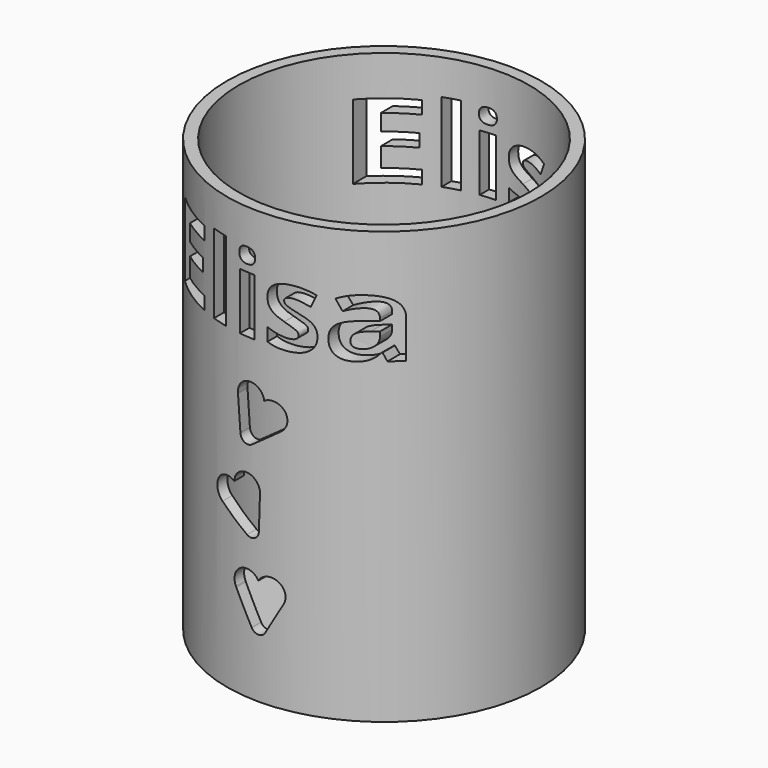
from build123d import *

# Parameters (mm, degrees)
F0_R         = 40
F1_DEPTH     = 110
F2_R         = 37
F3_DEPTH     = 104
F4_TEXT_SIZE = 26.5376641327
F5_DEPTH     = 45
F6_DEPTH     = 45


# Not quite as in the source:
# - Text() gives the source's letters only with a copy of the font that has no kerning and outlines rounded to 1/6400 em; it was checked with that copy


with BuildPart() as f1:
    # F0 (on Top) → F1 (new body)
    with BuildSketch(Plane.XY):
        Circle(F0_R)
    extrude(amount=F1_DEPTH)

    # F2 (on face) → F3 (cut)
    with BuildSketch(Plane.XY.offset(110)):
        Circle(F2_R)
    extrude(amount=-F3_DEPTH, mode=Mode.SUBTRACT)

    # F4 (on Front) → F5 (cut, symmetric)
    with BuildSketch(Plane.XZ):
        with BuildLine():
            ThreePointArc((6.0980562795, 23.7189958695), (4.7163435964, 28.3977795102), (0, 27.1502822652))
            ThreePointArc((0, 27.1502822652), (-4.7163435964, 28.3977795102), (-6.0980562795, 23.7189958695))
            Line((-6.0980562795, 23.7189958695), (-5.9870867882, 23.523414382))
            Line((-5.9870867882, 23.523414382), (-1.7395100946, 16.03714624))
            ThreePointArc((-1.7395100946, 16.03714624), (-1.0064952106, 15.2958291084), (0, 15.024113631))
            ThreePointArc((0, 15.024113631), (1.0064952106, 15.2958291084), (1.7395100946, 16.03714624))
            Line((1.7395100946, 16.03714624), (5.9870867882, 23.523414382))
            Line((5.9870867882, 23.523414382), (6.0980562795, 23.7189958695))
        make_face()
        with BuildLine():
            Line((-5.9870867882, 23.523414382), (-6.0980562795, 23.7189958695))
            ThreePointArc((-6.0980562795, 23.7189958695), (-6.0441426655, 23.6203136933), (-5.9870867882, 23.523414382))
        make_face()
        with BuildLine():
            ThreePointArc((5.9870867882, 23.523414382), (6.0441426655, 23.6203136933), (6.0980562795, 23.7189958695))
            Line((6.0980562795, 23.7189958695), (5.9870867882, 23.523414382))
        make_face()
        with BuildLine():
            ThreePointArc((0.3949105078, 46.6853627057), (-2.8839636057, 50.4050689505), (-6.5919721438, 47.1129719469))
            ThreePointArc((-6.5919721438, 47.1129719469), (-11.4072011799, 45.9294182599), (-10.2065108138, 41.1184336783))
            Line((-10.2065108138, 41.1184336783), (-2.9654370981, 36.4651584979))
            ThreePointArc((-2.9654370981, 36.4651584979), (-1.9718103227, 36.1496149336), (-0.9543788911, 36.3769806997))
            ThreePointArc((-0.9543788911, 36.3769806997), (-0.1895946703, 37.0854769985), (0.1147386299, 38.0825944199))
            Line((0.1147386299, 38.0825944199), (0.3949105078, 46.6853627057))
        make_face()
        with BuildLine():
            ThreePointArc((5.5303396509, 62.2585198994), (6.255422096, 67.0828749592), (1.453748051, 67.9454714242))
            ThreePointArc((1.453748051, 67.9454714242), (-2.2934957595, 71.0693008242), (-5.523092133, 67.4128197891))
            Line((-5.523092133, 67.4128197891), (-5.5051759271, 67.1886650304))
            Line((-5.5051759271, 67.1886650304), (-4.8193977228, 58.6086984387))
            ThreePointArc((-4.8193977228, 58.6086984387), (-4.468354783, 57.6270514736), (-3.6709922587, 56.9554303641))
            ThreePointArc((-3.6709922587, 56.9554303641), (-2.643965889, 56.7763249608), (-1.6663346341, 57.1384009738))
            Line((-1.6663346341, 57.1384009738), (5.3471108284, 62.1281606078))
            Line((5.3471108284, 62.1281606078), (5.5303396509, 62.2585198994))
        make_face()
        with BuildLine():
            Line((-5.5051759271, 67.1886650304), (-5.523092133, 67.4128197891))
            ThreePointArc((-5.523092133, 67.4128197891), (-5.5159346946, 67.3005984865), (-5.5051759271, 67.1886650304))
        make_face()
        with BuildLine():
            ThreePointArc((5.3471108284, 62.1281606078), (5.4397724329, 62.1918683525), (5.5303396509, 62.2585198994))
            Line((5.5303396509, 62.2585198994), (5.3471108284, 62.1281606078))
        make_face()
        with Locations((-30, 80.8928818245)):
            Text('Elisa', F4_TEXT_SIZE, font='Open Sans', font_style=FontStyle.BOLD, text_align=(TextAlign.LEFT, TextAlign.BOTTOM))
    extrude(amount=F5_DEPTH, both=True, mode=Mode.SUBTRACT)

    # F4 (on Front) → F6 (cut, symmetric)
    with BuildSketch(Plane.XZ):
        with BuildLine():
            ThreePointArc((6.0980562795, 23.7189958695), (4.7163435964, 28.3977795102), (0, 27.1502822652))
            ThreePointArc((0, 27.1502822652), (-4.7163435964, 28.3977795102), (-6.0980562795, 23.7189958695))
            Line((-6.0980562795, 23.7189958695), (-5.9870867882, 23.523414382))
            Line((-5.9870867882, 23.523414382), (-1.7395100946, 16.03714624))
            ThreePointArc((-1.7395100946, 16.03714624), (-1.0064952106, 15.2958291084), (0, 15.024113631))
            ThreePointArc((0, 15.024113631), (1.0064952106, 15.2958291084), (1.7395100946, 16.03714624))
            Line((1.7395100946, 16.03714624), (5.9870867882, 23.523414382))
            Line((5.9870867882, 23.523414382), (6.0980562795, 23.7189958695))
        make_face()
        with BuildLine():
            ThreePointArc((5.9870867882, 23.523414382), (6.0441426655, 23.6203136933), (6.0980562795, 23.7189958695))
            Line((6.0980562795, 23.7189958695), (5.9870867882, 23.523414382))
        make_face()
        with BuildLine():
            ThreePointArc((0.3949105078, 46.6853627057), (-2.8839636057, 50.4050689505), (-6.5919721438, 47.1129719469))
            ThreePointArc((-6.5919721438, 47.1129719469), (-11.4072011799, 45.9294182599), (-10.2065108138, 41.1184336783))
            Line((-10.2065108138, 41.1184336783), (-2.9654370981, 36.4651584979))
            ThreePointArc((-2.9654370981, 36.4651584979), (-1.9718103227, 36.1496149336), (-0.9543788911, 36.3769806997))
            ThreePointArc((-0.9543788911, 36.3769806997), (-0.1895946703, 37.0854769985), (0.1147386299, 38.0825944199))
            Line((0.1147386299, 38.0825944199), (0.3949105078, 46.6853627057))
        make_face()
        with Locations((-30, 80.8928818245)):
            Text('Elisa', F4_TEXT_SIZE, font='Open Sans', font_style=FontStyle.BOLD, text_align=(TextAlign.LEFT, TextAlign.BOTTOM))
    extrude(amount=F6_DEPTH, both=True, mode=Mode.SUBTRACT)


solid = f1.part
